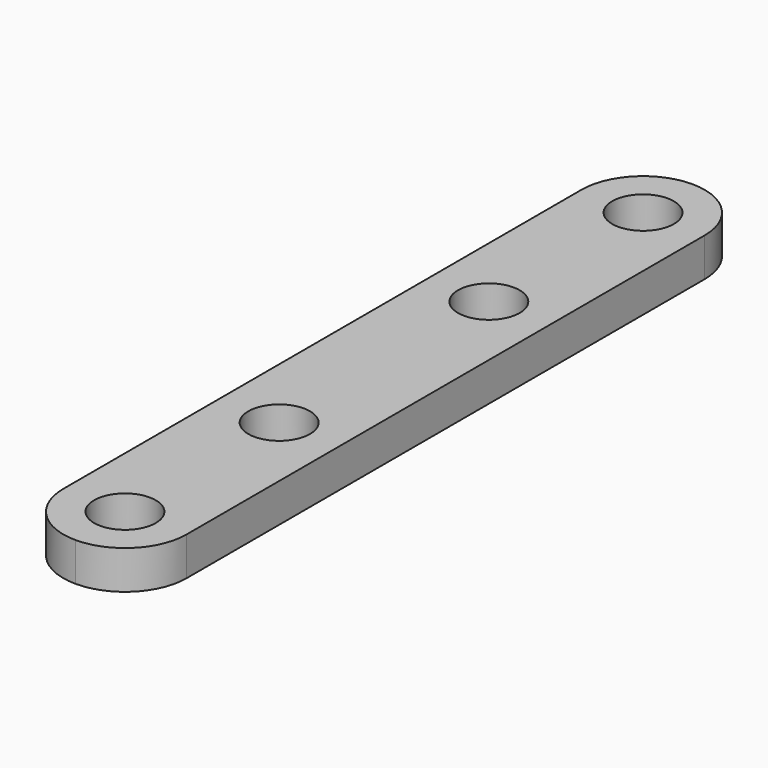
from build123d import *

# Parameters (mm, degrees)
F0_W     = 16
F0_H     = 100
F1_DEPTH = 5
F2_R     = 7.99999
F4_D     = 8


# Not quite as in the source:
# - a fillet or chamfer is up to 0.001 mm smaller than in the source, because OpenCascade refuses the exact size


with BuildPart() as f1:
    # F0 (on Top) → F1 (new body)
    with BuildSketch(Plane.XY):
        with Locations((8, 50)):
            Rectangle(F0_W, F0_H)
    extrude(amount=F1_DEPTH)

    # F2 (radius 8 in the source; OpenCascade refuses exactly that, so slightly less here)
    f2_edges = [f1.edges().sort_by_distance(p)[0] for p in [
        (16, 0, 2.5),
        (0, 0, 2.5),
        (16, 100, 2.5),
        (0, 100, 2.5),
    ]]
    fillet(f2_edges, radius=F2_R)

    # F4 (through all)
    with Locations(Plane.XY.offset(5)):
        with Locations((8, 92), (8, 67), (8, 33), (8, 8)):
            Hole(F4_D / 2)


solid = f1.part
